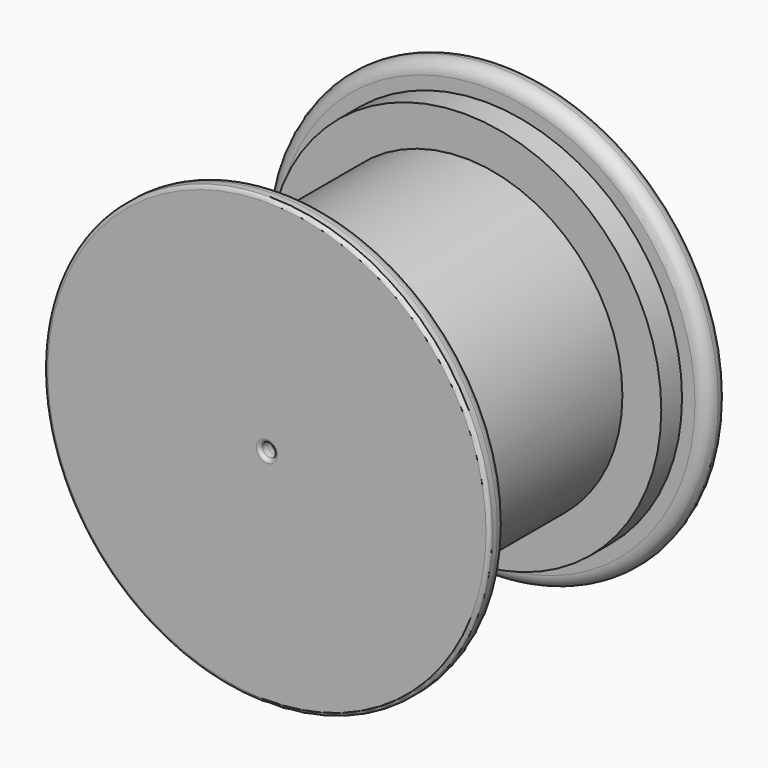
from build123d import *

# Parameters (mm, degrees)
F0_W = 42.1716768198
F0_H = 99.2274731398


with BuildPart() as f1:
    # F0 (on Top) → F1 (revolve)
    with BuildSketch(Plane.XY):
        Polygon((-44.3906867288, 47.101650387), (-25.3406867288, 47.101650387), (16.830990091, 47.101650387), (35.880990091, 47.101650387), (35.880990091, 59.801650387), (-44.3906867288, 59.801650387), align=None)
        with Locations((-4.2548483189, -2.5120861828)):
            Rectangle(F0_W, F0_H)
        Polygon((16.830990091, -52.1258227527), (-25.3406867288, -52.1258227527), (-38.0406867288, -52.1258227527), (-38.0406867288, -62.9278048873), (29.530990091, -62.9278048873), (29.530990091, -52.1258227527), align=None)
        with BuildLine():
            Line((-50.7406867288, 59.801650387), (-44.3906867288, 59.801650387))
            Line((-44.3906867288, 59.801650387), (35.880990091, 59.801650387))
            Line((35.880990091, 59.801650387), (42.230990091, 59.801650387))
            ThreePointArc((42.230990091, 59.801650387), (46.7211181515, 61.6615223265), (48.580990091, 66.151650387))
            ThreePointArc((48.580990091, 66.151650387), (46.7211181515, 70.6417784476), (42.230990091, 72.501650387))
            Line((42.230990091, 72.501650387), (-50.7406867288, 72.501650387))
            ThreePointArc((-50.7406867288, 72.501650387), (-55.2308147893, 70.6417784476), (-57.0906867288, 66.151650387))
            ThreePointArc((-57.0906867288, 66.151650387), (-55.2308147893, 61.6615223265), (-50.7406867288, 59.801650387))
        make_face()
        with BuildLine():
            Line((29.530990091, -62.9278048873), (-38.0406867288, -62.9278048873))
            Line((-38.0406867288, -62.9278048873), (-50.7406867288, -62.9278048873))
            ThreePointArc((-50.7406867288, -62.9278048873), (-55.2308147893, -64.7876768268), (-57.0906867288, -69.2778048873))
            Line((-57.0906867288, -69.2778048873), (-57.0906867288, -72.2609122954))
            ThreePointArc((-57.0906867288, -72.2609122954), (-56.5868863087, -73.4771941024), (-55.3706045017, -73.9809945226))
            Line((-55.3706045017, -73.9809945226), (46.8609078638, -73.9809945226))
            ThreePointArc((46.8609078638, -73.9809945226), (48.0771896708, -73.4771941024), (48.580990091, -72.2609122954))
            Line((48.580990091, -72.2609122954), (48.580990091, -69.2778048873))
            ThreePointArc((48.580990091, -69.2778048873), (46.7211181515, -64.7876768268), (42.230990091, -62.9278048873))
            Line((42.230990091, -62.9278048873), (29.530990091, -62.9278048873))
        make_face()
    revolve(axis=Axis((-60.5413205922, 7.4106594548, 0), (0, -1, 0)))


solid = f1.part
